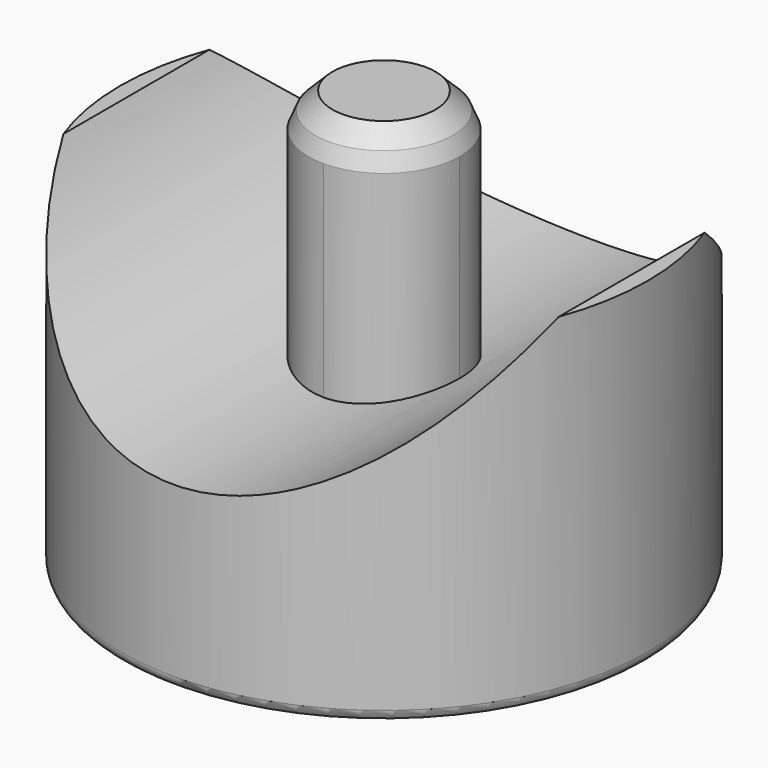
from build123d import *

# Parameters (mm, degrees)
F0_R     = 11
F1_DEPTH = 14.1
F2_R     = 11.385
F3_DEPTH = 28.4
F5_DEPTH = 17.5
F7_R     = 0.4828427125


# Not quite as in the source:
# - a fillet or chamfer that OpenCascade refuses, or shapes differently, is made with other operations: its cross-section is extruded or revolved along the edge and cut away or added


with BuildPart() as f1:
    # F0 (on Top) → F1 (new body)
    with BuildSketch(Plane.XY):
        with Locations((0, -12.3603016903)):
            Circle(F0_R)
    extrude(amount=F1_DEPTH)

    # F2 (on Front) → F3 (cut)
    with BuildSketch(Plane.XZ):
        with Locations((0, 18.905)):
            Circle(F2_R)
    extrude(amount=F3_DEPTH, mode=Mode.SUBTRACT)

    # F4 (on face) → F5 (join)
    with BuildSketch(Plane(origin=(0, 0, 0), x_dir=(1, 0, 0), z_dir=(0, 0, -1))):
        with BuildLine():
            ThreePointArc((0, 15.5053016903), (-3.145, 12.3603016903), (0, 9.2153016903))
            Line((0, 9.2153016903), (0, 15.5053016903))
        make_face()
        with BuildLine():
            Line((0, 15.5053016903), (0, 9.2153016903))
            ThreePointArc((0, 9.2153016903), (2.2238508268, 10.1364508634), (3.145, 12.3603016903))
            ThreePointArc((3.145, 12.3603016903), (2.2238508268, 14.5841525171), (0, 15.5053016903))
        make_face()
    extrude(amount=-F5_DEPTH)

    # F6: chamfer of 1 on 1 edges, made by hand

    # F6_s1 → F6_t2 (revolve, cut)
    with BuildSketch(Plane.YZ):
        Polygon((-9.2153016903, 16.5), (-10.2153016903, 17.5), (-9.2153016903, 17.5), align=None)
    revolve(axis=Axis((0, -12.3603016903, 17.5), (0, 0, -1)), mode=Mode.SUBTRACT)

    # F7
    f7_edges = [f1.edges().sort_by_distance(p)[0] for p in [
        (-11, -12.360302, 0),
    ]]
    fillet(f7_edges, radius=F7_R)

    # F8: chamfer of 0.4 on 1 edges, made by hand

    # F8_s1 → F8_t2 (revolve, cut)
    with BuildSketch(Plane.YZ):
        Polygon((-9.2153016903, 16.1), (-9.4981444028, 16.7828427125), (-9.2153016903, 16.5), align=None)
    revolve(axis=Axis((0, -12.3603016903, 16.5), (0, 0, -1)), mode=Mode.SUBTRACT)


solid = f1.part
